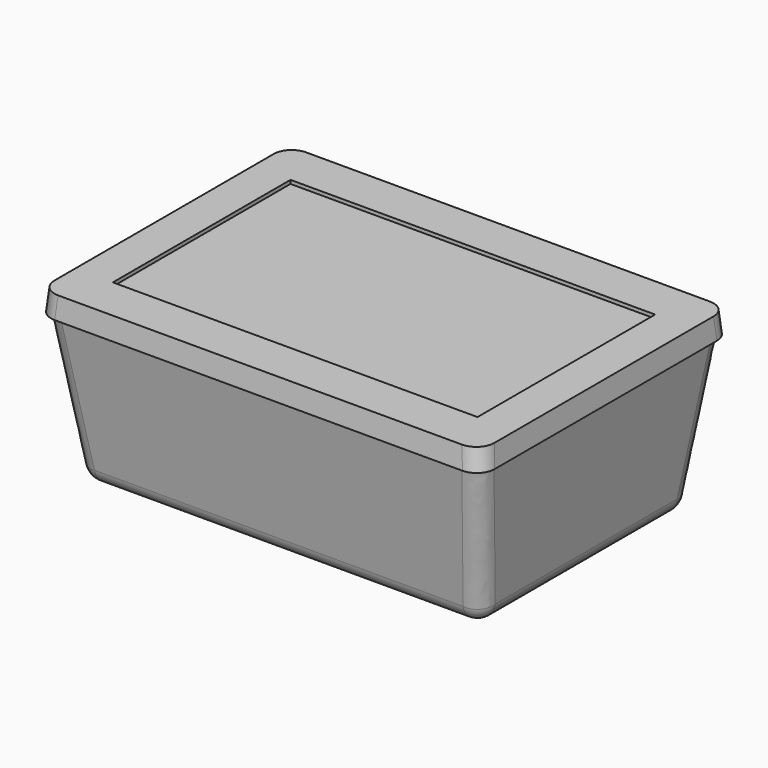
from build123d import *

# Parameters (mm, degrees)
F0_W        = 111.22
F0_H        = 71.63
F2_W        = 121.14
F2_H        = 85.07
F4_R        = 5
F6_W        = 123.14
F6_H        = 87.07
F7_DEPTH    = 6
F8_T1_DEPTH = 154.335608958
F8_T3_DEPTH = 118.265608958
F10_W       = 101.22
F10_H       = 61.63
F11_DEPTH   = 1
F12_R       = 5


# Not quite as in the source:
# - a fillet or chamfer that OpenCascade refuses, or shapes differently, is made with other operations: its cross-section is extruded or revolved along the edge and cut away or added


with BuildPart() as f3:
    # F0 (on Top) → F3 section 0
    with BuildSketch(Plane.XY):
        Rectangle(F0_W, F0_H)
    # F2 (on offset) → F3 section 1
    with BuildSketch(Plane.XY.offset(42)):
        Rectangle(F2_W, F2_H)
    loft()

    # F4
    f4_edges = [f3.edges().sort_by_distance(p)[0] for p in [
        (-58.09, -39.175, 21),
        (0, -35.815, 0),
        (58.09, -39.175, 21),
        (55.61, 0, 0),
        (58.09, 39.175, 21),
        (0, 35.815, 0),
        (-58.09, 39.175, 21),
        (-55.61, 0, 0),
    ]]
    fillet(f4_edges, radius=F4_R)

    # F6 (on offset) → F7 (join)
    with BuildSketch(Plane.XY.offset(42)):
        Rectangle(F6_W, F6_H)
    extrude(amount=F7_DEPTH)

    # F8: chamfer of 6 x 0.5249319812 on 4 edges, made by hand

    # F8_s2 → F8_t1 (cut)
    with BuildSketch(Plane.YZ.offset(-77.167804479)):
        Polygon((-43.535, 42), (-43.0100680188, 48), (-43.535, 48), align=None)
        Polygon((43.535, 42), (43.0100680188, 48), (43.535, 48), align=None)
    extrude(amount=F8_T1_DEPTH, mode=Mode.SUBTRACT)

    # F8_s4 → F8_t3 (cut)
    with BuildSketch(Plane.XZ.offset(-59.132804479)):
        Polygon((-61.0450680188, 48), (-61.57, 42), (-61.57, 48), align=None)
        Polygon((61.57, 42), (61.0450680188, 48), (61.57, 48), align=None)
    extrude(amount=F8_T3_DEPTH, mode=Mode.SUBTRACT)

    # F10 (on offset) → F11 (cut)
    with BuildSketch(Plane.XY.offset(48)):
        Rectangle(F10_W, F10_H)
    extrude(amount=-F11_DEPTH, mode=Mode.SUBTRACT)

    # F12
    f12_edges = [f3.edges().sort_by_distance(p)[0] for p in [
        (-61.307534, -43.272534, 45),
        (61.307534, -43.272534, 45),
        (61.307534, 43.272534, 45),
        (-61.307534, 43.272534, 45),
    ]]
    fillet(f12_edges, radius=F12_R)


solid = f3.part
